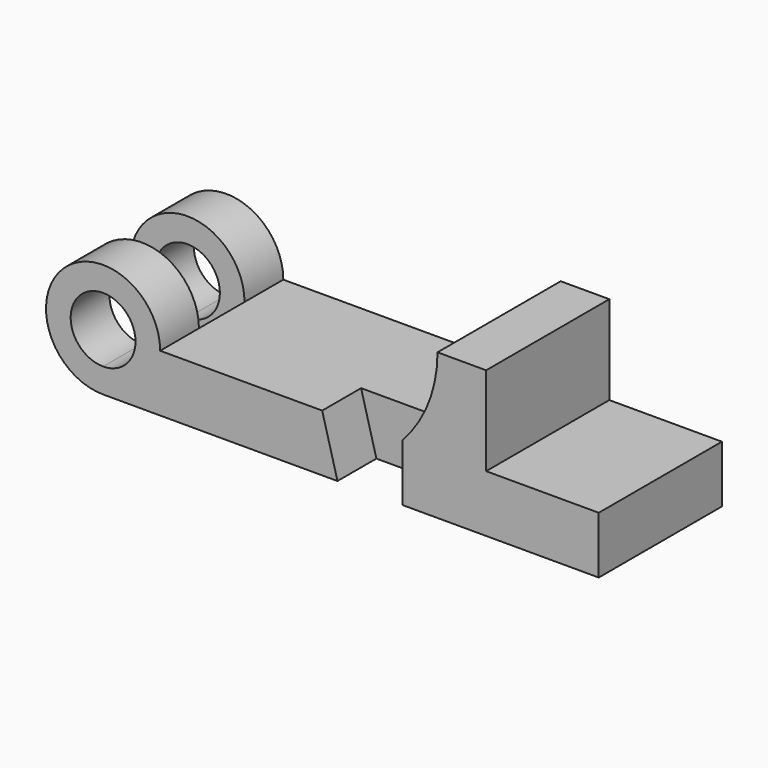
from build123d import *

# Parameters (mm, degrees)
F0_W     = 19.05
F0_H     = 34.798
F1_DEPTH = 30.1625
F3_DEPTH = 19.05
F5_W     = 44.704
F5_H     = 22.3266
F6_DEPTH = 49.531


with BuildPart() as f1:
    # F0 (on Front) → F1 (new body, symmetric)
    with BuildSketch(Plane.XZ):
        Polygon((97.1042, 0), (97.1042, 22.352), (52.9844, 22.352), (33.9344, 22.352), (20.1443877871, 22.352), (20.1443877871, 0), align=None)
        with Locations((43.4594, 39.751)):
            Rectangle(F0_W, F0_H)
        with BuildLine():
            Line((20.1443877871, 22.352), (33.9344, 22.352))
            Line((33.9344, 22.352), (33.9344, 57.15))
            ThreePointArc((33.9344, 57.15), (30.3612323074, 38.4345969798), (20.1443877871, 22.352))
        make_face()
        with BuildLine():
            Line((-97.1042, 0), (20.1443877871, 0))
            Line((20.1443877871, 0), (20.1443877871, 22.352))
            Line((20.1443877871, 22.352), (-74.7522, 22.352))
            ThreePointArc((-74.7522, 22.352), (-81.2989492269, 6.5467492269), (-97.1042, 0))
        make_face()
        with BuildLine():
            ThreePointArc((-74.7522, 22.352), (-112.9094507731, 38.1572507731), (-97.1042, 0))
            Line((-97.1042, 0), (-97.1042, 9.652))
            ThreePointArc((-97.1042, 9.652), (-106.0844561211, 31.3322561211), (-84.4042, 22.352))
            Line((-84.4042, 22.352), (-74.7522, 22.352))
        make_face()
        with BuildLine():
            Line((-97.1042, 9.652), (-97.1042, 0))
            ThreePointArc((-97.1042, 0), (-81.2989492269, 6.5467492269), (-74.7522, 22.352))
            Line((-74.7522, 22.352), (-84.4042, 22.352))
            ThreePointArc((-84.4042, 22.352), (-88.1239438789, 13.3717438789), (-97.1042, 9.652))
        make_face()
    extrude(amount=F1_DEPTH, both=True)

    # F2 (on face) → F3 (cut)
    with BuildSketch(Plane.XZ.offset(30.1625)):
        Polygon((-5.2578, 0), (20.1443877871, 0), (20.1443877871, 22.352), (-11.2522, 22.352), align=None)
    extrude(amount=-F3_DEPTH, mode=Mode.SUBTRACT)

    # F5 (on offset) → F6 (cut, through all)
    with BuildSketch(Plane.XY.offset(49.53)):
        with Locations((-97.1042, 0)):
            Rectangle(F5_W, F5_H)
    extrude(amount=-F6_DEPTH, mode=Mode.SUBTRACT)


solid = f1.part
